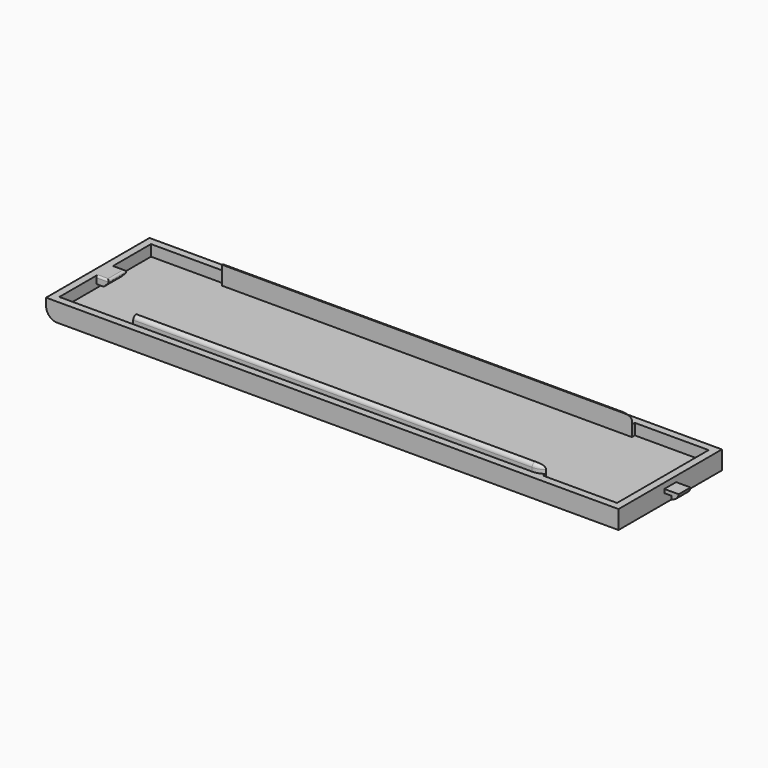
from build123d import *

# Parameters (mm, degrees)
F0_W         = 35
F0_H         = 5
F1_DEPTH     = 77.5
F2_T         = -2
F4_DEPTH     = 3
F6_DEPTH     = 2
F7_T1_DEPTH  = 10.0971618345
F8_W         = 111
F8_H         = 5
F9_DEPTH     = 1
F10_W        = 111
F10_H        = 2
F10_H_2      = 3
F11_DEPTH    = 1
F12_T1_DEPTH = 9.5
F13_R        = 0.99999
F14_R        = 0.5
F15_R        = 4
F16_DEPTH    = 1
F17_W        = 2
F17_H        = 10
F18_DEPTH    = 1
F19_R        = 0.99999
F20_R        = 3


# Not quite as in the source:
# - a fillet or chamfer that OpenCascade refuses, or shapes differently, is made with other operations: its cross-section is extruded or revolved along the edge and cut away or added
# - a fillet or chamfer is up to 0.001 mm smaller than in the source, because OpenCascade refuses the exact size


with BuildPart() as f1:
    # F0 (on Right) → F1 (new body, symmetric)
    with BuildSketch(Plane.YZ):
        Rectangle(F0_W, F0_H)
    extrude(amount=F1_DEPTH, both=True)

    # F2
    f2_openings = [f1.faces().sort_by_distance(p)[0] for p in [
        (0, 0, 2.5),
    ]]
    offset(amount=F2_T, openings=f2_openings)

    # F3 (on Front) → F4 (join, symmetric)
    with BuildSketch(Plane.XZ):
        Polygon((-71.5, 2.5), (-75.5, 2.5), (-75.5, 0.5), (-73.5, 0.5), align=None)
    extrude(amount=F4_DEPTH, both=True)

    # F5 (on Front) → F6 (join, symmetric)
    with BuildSketch(Plane.XZ):
        Polygon((81.4, 1), (77.5, 1), (77.5, 0), (79.4, 0), (81.4, 0), align=None)
        Polygon((79.4, -1), (81.4, 0), (79.4, 0), align=None)
    extrude(amount=F6_DEPTH, both=True)

    # F7: fillet of radius 2 on 1 edges, made by hand

    # F7_s2 → F7_t1 (cut)
    with BuildSketch(Plane.XZ.offset(-5.0485809173)):
        with BuildLine():
            ThreePointArc((81.4, 1), (81.0488845703, 0.09023972), (80.3093065335, -0.5453467333))
            Line((80.3093065335, -0.5453467333), (81.4, 0))
            Line((81.4, 0), (81.4, 1))
        make_face()
    extrude(amount=F7_T1_DEPTH, mode=Mode.SUBTRACT)

    # F8 (on face) → F9 (join)
    with BuildSketch(Plane(origin=(0, -15.5, 0), x_dir=(-1, 0, 0), z_dir=(0, 1, 0))):
        with Locations((0, 2)):
            Rectangle(F8_W, F8_H)
    extrude(amount=F9_DEPTH)

    # F10 (on face) → F11 (join)
    with BuildSketch(Plane.XZ.offset(-15.5)):
        with Locations((0, 3.5)):
            Rectangle(F10_W, F10_H)
        with Locations((0, 1)):
            Rectangle(F10_W, F10_H_2)
    extrude(amount=F11_DEPTH)

    # F12: fillet of radius 5 on 2 edges, made by hand

    # F12_s2 → F12_t1 (cut)
    with BuildSketch(Plane.XY.offset(2.5)):
        with BuildLine():
            ThreePointArc((52.5, 15.5), (54.0811388301, 15.2434164903), (55.5, 14.5))
            Line((55.5, 14.5), (55.5, 15.5))
            Line((55.5, 15.5), (52.5, 15.5))
        make_face()
        with BuildLine():
            ThreePointArc((52.5, -15.5), (54.0811388301, -15.2434164903), (55.5, -14.5))
            Line((55.5, -14.5), (55.5, -15.5))
            Line((55.5, -15.5), (52.5, -15.5))
        make_face()
    extrude(amount=F12_T1_DEPTH, mode=Mode.SUBTRACT)

    # F13 (radius 1 in the source; OpenCascade refuses exactly that, so slightly less here)
    f13_edges = [f1.edges().sort_by_distance(p)[0] for p in [
        (-1.5, -15.5, 4.5),
        (-1.5, 15.5, 4.5),
    ]]
    fillet(f13_edges, radius=F13_R)

    # F14
    f14_edges = [f1.edges().sort_by_distance(p)[0] for p in [
        (-71.5, 0, 2.5),
        (-73.5, -3, 2.5),
        (-73.5, 3, 2.5),
    ]]
    fillet(f14_edges, radius=F14_R)

    # F15 (on face) → F16 (cut)
    with BuildSketch(Plane(origin=(0, 0, -2.5), x_dir=(1, 0, 0), z_dir=(0, 0, -1))):
        with Locations((-64.5, 11.5)):
            Circle(F15_R)
        with Locations((-64.5, -11.5)):
            Circle(F15_R)
        with Locations((69.5, -11.5)):
            Circle(F15_R)
        with Locations((69.5, 11.5)):
            Circle(F15_R)
    extrude(amount=-F16_DEPTH, mode=Mode.SUBTRACT)

    # F17 (on face) → F18 (join)
    with BuildSketch(Plane(origin=(0, 0, -2.5), x_dir=(1, 0, 0), z_dir=(0, 0, -1))):
        with Locations((71.5, 0)):
            Rectangle(F17_W, F17_H)
    extrude(amount=F18_DEPTH)

    # F19 (radius 1 in the source; OpenCascade refuses exactly that, so slightly less here)
    f19_edges = [f1.edges().sort_by_distance(p)[0] for p in [
        (71.5, -5, -3.5),
        (72.5, 0, -3.5),
        (71.5, 5, -3.5),
        (70.5, 0, -3.5),
    ]]
    fillet(f19_edges, radius=F19_R)

    # F20
    f20_edges = [f1.edges().sort_by_distance(p)[0] for p in [
        (-77.5, 0, -2.5),
    ]]
    fillet(f20_edges, radius=F20_R)


solid = f1.part
